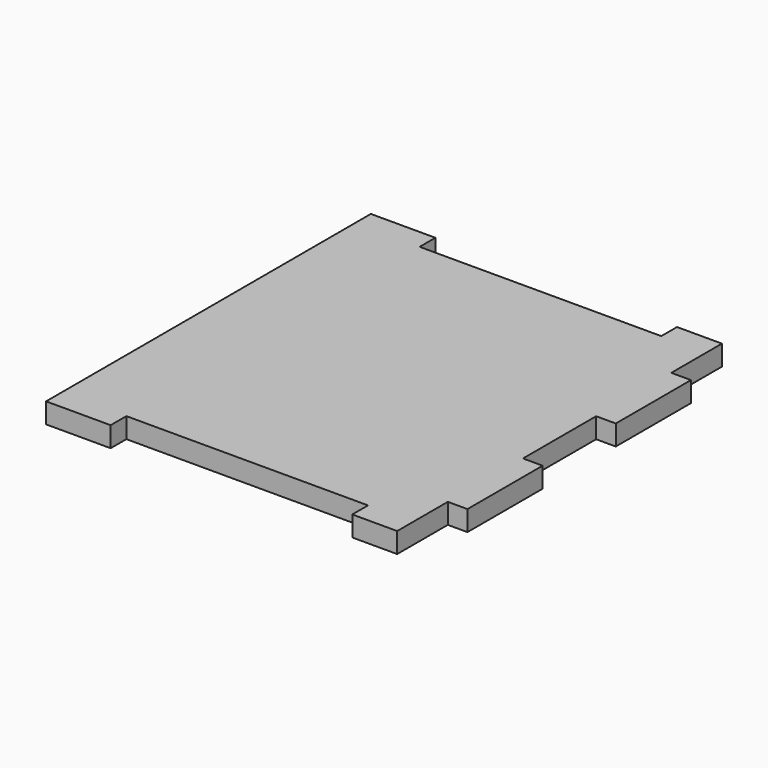
from build123d import *

# Parameters (mm, degrees)
F0_W     = 58
F0_H     = 63.5
F1_DEPTH = 3.175
F2_W     = 37.8
F2_H     = 3.075
F2_W_2   = 3.075
F2_H_2   = 14.3
F2_H_3   = 9.9
F3_DEPTH = 25


# Not quite as in the source:
# - a length typed as a fraction of an inch, garbled in the dataset ("3 / 203.2 mm" for 3/8 in), is restored


with BuildPart() as f1:
    # F0 (on Top) → F1 (new body)
    with BuildSketch(Plane.XY):
        Rectangle(F0_W, F0_H)
    extrude(amount=F1_DEPTH)

    # F2 (on face) → F3 (cut)
    with BuildSketch(Plane.XY.offset(3.175)):
        with Locations((0, -30.2125)):
            Rectangle(F2_W, F2_H)
        with Locations((0, 30.2125)):
            Rectangle(F2_W, F2_H)
        with Locations((27.4625, 0)):
            Rectangle(F2_W_2, F2_H_2)
        with Locations((27.4625, -26.8)):
            Rectangle(F2_W_2, F2_H_3)
        with Locations((27.4625, 26.8)):
            Rectangle(F2_W_2, F2_H_3)
    extrude(amount=-F3_DEPTH, mode=Mode.SUBTRACT)


solid = f1.part
